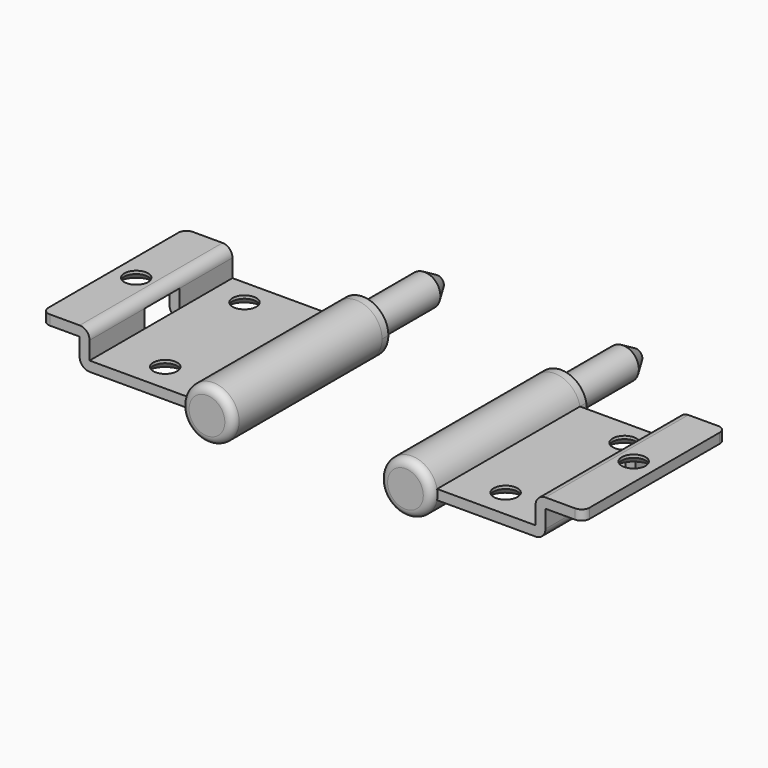
from build123d import *

# Parameters (mm, degrees)
F1_DEPTH        = 45
F2_R            = 2
F3_R            = 2.5
F5_DEPTH        = 2
F6_R            = 4
F7_DEPTH        = 23.5
F8_SIZE2        = 2.31
F8_SIZE         = 4
F10_D           = 6
F10_CSINK_D     = 9.5
F10_CSINK_ANGLE = 90
F11_R           = 6.5
F12_DEPTH       = 2
F14_W           = 5
F14_H           = 11
F15_DEPTH       = 25
F16_D           = 6
F16_CSINK_D     = 9.5
F16_CSINK_ANGLE = 90


# Not quite as in the source:
# - a fillet or chamfer that OpenCascade refuses, or shapes differently, is made with other operations: its cross-section is extruded or revolved along the edge and cut away or added
# - a feature names something its author has since deleted; it is built from what else it names


with BuildPart() as f1:
    # F0 (on Front) → F1 (new body)
    with BuildSketch(Plane.XZ):
        with BuildLine():
            Line((31.1786754111, 1.25), (6.3786754111, 1.25))
            ThreePointArc((6.3786754111, 1.25), (-6.5, 0), (6.3786754111, -1.25))
            Line((6.3786754111, -1.25), (33.6786754111, -1.25))
            Line((33.6786754111, -1.25), (33.6786754111, 5.75))
            Line((33.6786754111, 5.75), (43.1786754111, 5.75))
            Line((43.1786754111, 5.75), (43.1786754111, 8.25))
            Line((43.1786754111, 8.25), (31.1786754111, 8.25))
            Line((31.1786754111, 8.25), (31.1786754111, 1.25))
        make_face()
    extrude(amount=F1_DEPTH)

    # F2
    f2_edges = [f1.edges().sort_by_distance(p)[0] for p in [
        (43.178675, -45, 7),
        (43.178675, 0, 7),
    ]]
    fillet(f2_edges, radius=F2_R)

    # F3
    f3_edges = [f1.edges().sort_by_distance(p)[0] for p in [
        (33.678675, -22.5, -1.25),
        (31.178675, -22.5, 8.25),
    ]]
    fillet(f3_edges, radius=F3_R)

    # F4 (on face) → F5 (join)
    with BuildSketch(Plane(origin=(0, 0, 0), x_dir=(-1, 0, 0), z_dir=(0, 1, 0))):
        with BuildLine():
            ThreePointArc((-6.3786754111, -1.25), (0.6279370303, -6.469597753), (6.5, 0))
            ThreePointArc((6.5, 0), (0.6279370303, 6.469597753), (-6.3786754111, 1.25))
            ThreePointArc((-6.3786754111, 1.25), (-6.5, 0), (-6.3786754111, -1.25))
        make_face()
    extrude(amount=F5_DEPTH)

    # F6 (on face) → F7 (join)
    with BuildSketch(Plane(origin=(0, 2, 0), x_dir=(-1, 0, 0), z_dir=(0, 1, 0))):
        Circle(F6_R)
    extrude(amount=F7_DEPTH)

    # F8
    f8_edges = [f1.edges().sort_by_distance(p)[0] for p in [
        (4, 25.5, 0),
    ]]
    f8_side = f1.faces().sort_by_distance((4, 13.75, 0))[0]
    chamfer(f8_edges, length=F8_SIZE, length2=F8_SIZE2, reference=f8_side)

    # F10 (through all)
    with Locations(Plane(origin=(0, 0, -1.25), x_dir=(1, 0, 0), z_dir=(0, 0, -1))):
        with Locations((22.8786754111, 6.6), (17.8786754111, 37.8)):
            CounterSinkHole(F10_D / 2, F10_CSINK_D / 2, counter_sink_angle=F10_CSINK_ANGLE)

    # F11 (on face) → F12 (join)
    with BuildSketch(Plane.XZ.offset(45)):
        Circle(F11_R)
    extrude(amount=F12_DEPTH)

    # F13: fillet of radius 2 on 1 edges, made by hand

    # F13_s1 → F13_t2 (revolve, cut)
    with BuildSketch(Plane.XY):
        with BuildLine():
            ThreePointArc((6.5, -45), (5.9142135624, -46.4142135624), (4.5, -47))
            Line((4.5, -47), (6.5, -47))
            Line((6.5, -47), (6.5, -45))
        make_face()
    revolve(axis=Axis((0, -47, 0), (0, -1, 0)), mode=Mode.SUBTRACT)

    # F14 (on face) → F15 (cut)
    with BuildSketch(Plane(origin=(0, 0, 5.75), x_dir=(1, 0, 0), z_dir=(0, 0, -1))):
        with Locations((33.6786754111, 22.2)):
            Rectangle(F14_W, F14_H)
    extrude(amount=F15_DEPTH, mode=Mode.SUBTRACT)

    # F16 (through all)
    with Locations(Plane(origin=(0, 0, 5.75), x_dir=(1, 0, 0), z_dir=(0, 0, -1))):
        with Locations((37.6786754111, 22.2)):
            CounterSinkHole(F16_D / 2, F16_CSINK_D / 2, counter_sink_angle=F16_CSINK_ANGLE)


with BuildPart() as f18_1:
    # F18: instance of F1
    add(f1.part.mirror(Plane.YZ.offset(-25)))


solid = Compound([f1.part, f18_1.part])
